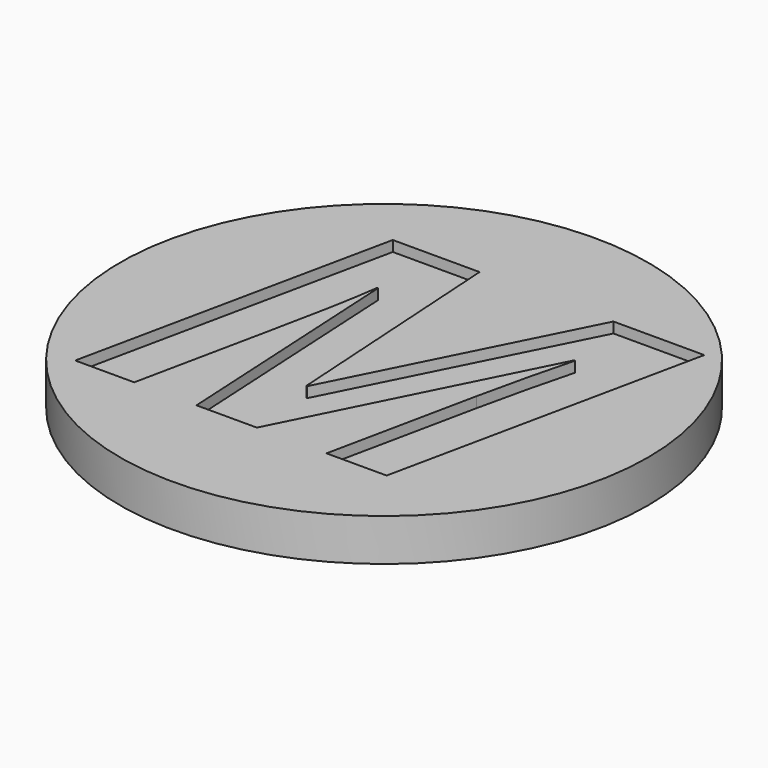
from build123d import *

# Parameters (mm, degrees)
F0_R         = 25
F1_DEPTH     = 4
F0_TEXT_SIZE = 41.6666666667
F2_DEPTH     = 3
F3_R         = 10.5
F4_DEPTH     = 2


# Not quite as in the source:
# - Text() gives the source's letters only with a copy of the font that has no kerning and outlines rounded to 1/6400 em; it was checked with that copy


with BuildPart() as f1:
    # F0 (on Top) → F1 (new body)
    with BuildSketch(Plane.XY):
        Circle(F0_R)
        with BuildLine():
            Line((-1.9026727297, -6.8307591726), (-1.818037313, -6.8307591726))
            Line((-1.818037313, -6.8307591726), (9.392900187, 15.4088241607))
            Line((9.392900187, 15.4088241607), (17.9996710203, 15.4088241607))
            Line((17.9996710203, 15.4088241607), (11.7106085203, -14.3372695893))
            Line((11.7106085203, -14.3372695893), (6.013993937, -14.3372695893))
            Line((6.013993937, -14.3372695893), (8.963212687, -0.2552383393))
            add(Edge.make_bspline(
                [(8.963212687, -0.2552383393), (10.0439418536, 4.7642929107), (11.0986293536, 8.7161158274)],
                knots=[0, 0, 0, 1, 1, 1], degree=2))
            Line((11.0986293536, 8.7161158274), (11.0009731036, 8.7161158274))
            Line((11.0009731036, 8.7161158274), (-0.5810581464, -14.3372695893))
            Line((-0.5810581464, -14.3372695893), (-6.2972039797, -14.3372695893))
            Line((-6.2972039797, -14.3372695893), (-7.5341831464, 8.7161158274))
            Line((-7.5341831464, 8.7161158274), (-7.618818563, 8.7161158274))
            add(Edge.make_bspline(
                [(-7.618818563, 8.7161158274), (-7.8401727297, 6.925751244), (-8.390302938, 4.015594994)],
                knots=[0, 0, 0, 1, 1, 1], degree=2))
            add(Edge.make_bspline(
                [(-8.390302938, 4.015594994), (-8.9404331464, 1.105438744), (-12.1956414797, -14.3372695893)],
                knots=[0, 0, 0, 1, 1, 1], degree=2))
            Line((-12.1956414797, -14.3372695893), (-17.7880893964, -14.3372695893))
            Line((-17.7880893964, -14.3372695893), (-11.505537313, 15.4088241607))
            Line((-11.505537313, 15.4088241607), (-3.282881063, 15.4088241607))
            Line((-3.282881063, 15.4088241607), (-1.9026727297, -6.8307591726))
        make_face(mode=Mode.SUBTRACT)
    extrude(amount=F1_DEPTH)

    # F0 (on Top) → F2 (join)
    with BuildSketch(Plane.XY):
        with Locations((-18.868818563, -14.3372695893)):
            Text('M', F0_TEXT_SIZE, font='Open Sans', font_style=FontStyle.BOLDITALIC, text_align=(TextAlign.LEFT, TextAlign.BOTTOM))
    extrude(amount=F2_DEPTH)

    # F3 (on face) → F4 (cut)
    with BuildSketch(Plane(origin=(0, 0, 0), x_dir=(1, 0, 0), z_dir=(0, 0, -1))):
        Circle(F3_R)
    extrude(amount=-F4_DEPTH, mode=Mode.SUBTRACT)


solid = f1.part
